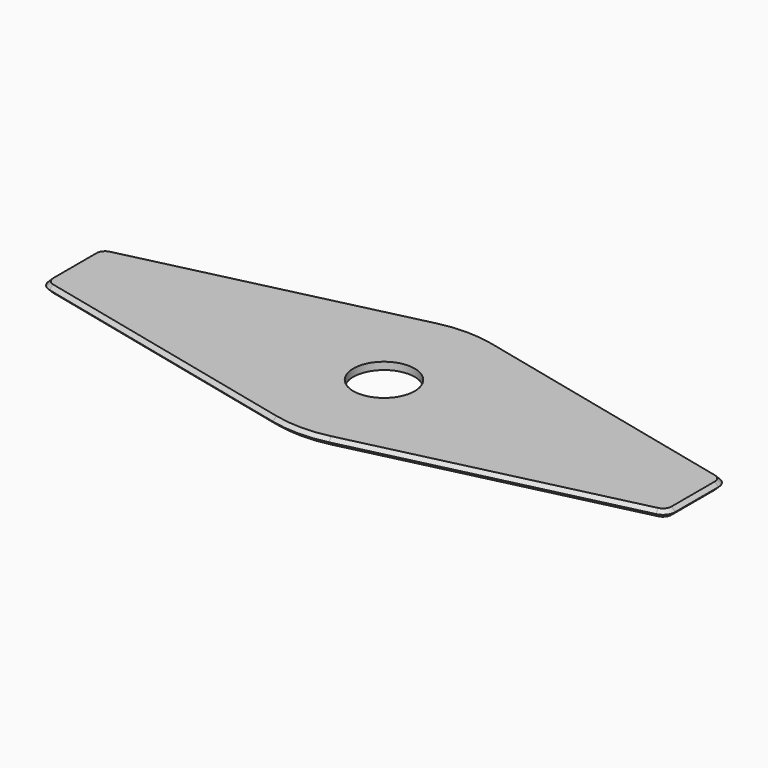
from build123d import *

# Parameters (mm, degrees)
F0_R     = 12.5
F1_DEPTH = 3
F2_R     = 50
F3_R     = 5
F4_SIZE  = 1.49999


# Not quite as in the source:
# - a fillet or chamfer is up to 0.001 mm smaller than in the source, because OpenCascade refuses the exact size


with BuildPart() as f1:
    # F0 (on Top) → F1 (new body)
    with BuildSketch(Plane.XY):
        Polygon((127.5, 15), (0, 45), (-127.5, 15), (-127.5, -15), (0, -45), (127.5, -15), align=None)
        Circle(F0_R, mode=Mode.SUBTRACT)
    extrude(amount=F1_DEPTH)

    # F2
    f2_edges = [f1.edges().sort_by_distance(p)[0] for p in [
        (0, 45, 1.5),
        (0, -45, 1.5),
    ]]
    fillet(f2_edges, radius=F2_R)

    # F3
    f3_edges = [f1.edges().sort_by_distance(p)[0] for p in [
        (127.5, 15, 1.5),
        (127.5, -15, 1.5),
        (-127.5, 15, 1.5),
        (-127.5, -15, 1.5),
    ]]
    fillet(f3_edges, radius=F3_R)

    # F4 (size 1.5 in the source; OpenCascade refuses exactly that, so slightly less here)
    f4_edges = [f1.edges().sort_by_distance(p)[0] for p in [
        (-67.548582, 29.106216, 3),
        (-67.548582, 29.106216, 0),
    ]]
    chamfer(f4_edges, length=F4_SIZE)


solid = f1.part
